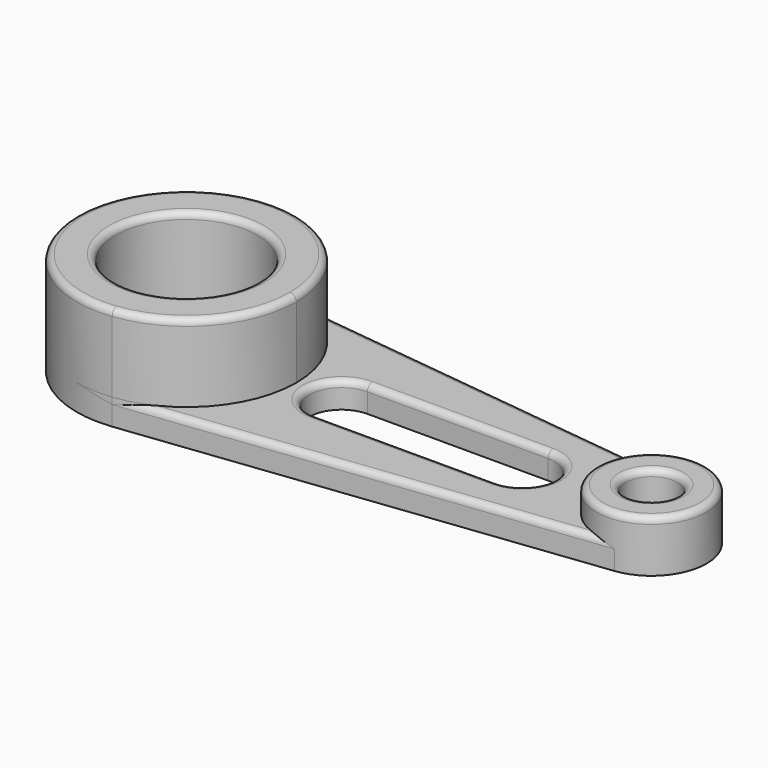
from build123d import *

# Parameters (mm, degrees)
F0_R         = 34.925
F1_DEPTH     = 50.8
F2_DEPTH     = 12.7
F0_R_2       = 12.7
F3_DEPTH     = 25.4
F4_F1_R      = 3.175
F4_F2_R      = 3.175
F4_F3_R      = 3.175
F4_F4_R      = 3.175
F4_F5_R      = 3.175
F4_T9_DEPTH  = 264.3151886434
F4_S10_R     = 27.051
F4_T11_DEPTH = 134
F4_S12_R     = 53.975
F4_T13_DEPTH = 134
F4_T17_DEPTH = 264.3151886434
F4_S18_R     = 27.051
F4_T19_DEPTH = 134
F4_S20_R     = 53.975
F4_T21_DEPTH = 134


# Not quite as in the source:
# - a fillet or chamfer that OpenCascade refuses, or shapes differently, is made with other operations: its cross-section is extruded or revolved along the edge and cut away or added


with BuildPart() as f1:
    # F0 (on Top) → F1 (new body)
    with BuildSketch(Plane.XY):
        with BuildLine():
            ThreePointArc((-174.625, 0), (-188.2488990323, 35.8481418723), (-222.2429444444, 53.5993327352))
            ThreePointArc((-222.2429444444, 53.5993327352), (-282.575, 0), (-222.2429444444, -53.5993327352))
            ThreePointArc((-222.2429444444, -53.5993327352), (-188.2488990323, -35.8481418723), (-174.625, 0))
        make_face()
        with Locations((-228.6, 0)):
            Circle(F0_R, mode=Mode.SUBTRACT)
    extrude(amount=F1_DEPTH)

    # F0 (on Top) → F2 (join)
    with BuildSketch(Plane.XY):
        with BuildLine():
            ThreePointArc((3.1860066667, -26.8627244061), (-27.051, 0), (3.1860066667, 26.8627244061))
            Line((3.1860066667, 26.8627244061), (-222.2429444444, 53.5993327352))
            ThreePointArc((-222.2429444444, 53.5993327352), (-188.2488990323, 35.8481418723), (-174.625, 0))
            ThreePointArc((-174.625, 0), (-188.2488990323, -35.8481418723), (-222.2429444444, -53.5993327352))
            Line((-222.2429444444, -53.5993327352), (3.1860066667, -26.8627244061))
        make_face()
        with BuildLine():
            ThreePointArc((-63.5, 15.875), (-52.2746798487, 11.2253201513), (-47.625, 0))
            ThreePointArc((-47.625, 0), (-52.2746798487, -11.2253201513), (-63.5, -15.875))
            Line((-63.5, -15.875), (-152.4, -15.875))
            ThreePointArc((-152.4, -15.875), (-168.275, 0), (-152.4, 15.875))
            Line((-152.4, 15.875), (-63.5, 15.875))
        make_face(mode=Mode.SUBTRACT)
    extrude(amount=F2_DEPTH)

    # F0 (on Top) → F3 (join)
    with BuildSketch(Plane.XY):
        with BuildLine():
            ThreePointArc((3.1860066667, -26.8627244061), (20.2230223673, -17.9662452207), (27.051, 0))
            ThreePointArc((27.051, 0), (20.2230223673, 17.9662452207), (3.1860066667, 26.8627244061))
            ThreePointArc((3.1860066667, 26.8627244061), (-27.051, 0), (3.1860066667, -26.8627244061))
        make_face()
        Circle(F0_R_2, mode=Mode.SUBTRACT)
    extrude(amount=F3_DEPTH)

    # F4: fillet of radius 3.175 on 10 edges, made by hand

    # F4_f1
    f4_f1_edges = [f1.edges().sort_by_distance(p)[0] for p in [
        (-234.9570555556, 53.5993327352, 50.8),
    ]]
    fillet(f4_f1_edges, radius=F4_F1_R)

    # F4_f2
    f4_f2_edges = [f1.edges().sort_by_distance(p)[0] for p in [
        (-47.625, 0, 12.7),
        (-107.95, -15.875, 12.7),
        (-168.275, 0, 12.7),
        (-107.95, 15.875, 12.7),
    ]]
    fillet(f4_f2_edges, radius=F4_F2_R)

    # F4_f3
    f4_f3_edges = [f1.edges().sort_by_distance(p)[0] for p in [
        (-263.525, 0, 50.8),
    ]]
    fillet(f4_f3_edges, radius=F4_F3_R)

    # F4_f4
    f4_f4_edges = [f1.edges().sort_by_distance(p)[0] for p in [
        (-3.1860066667, 26.8627244061, 25.4),
    ]]
    fillet(f4_f4_edges, radius=F4_F4_R)

    # F4_f5
    f4_f5_edges = [f1.edges().sort_by_distance(p)[0] for p in [
        (-12.7, 0, 25.4),
    ]]
    fillet(f4_f5_edges, radius=F4_F5_R)


with BuildPart() as f4_tool7:
    # F4_s8 → F4_t9 (new body)
    with BuildSketch(Plane(origin=(-249.0757155531, -29.5411916624, 0), x_dir=(0, 0, 1), z_dir=(0.9930399766, 0.1177777778, 0))):
        with BuildLine():
            ThreePointArc((12.7, 23.876), (11.7700640303, 26.1210640303), (9.525, 27.051))
            Line((9.525, 27.051), (9.525, 27.1145))
            Line((9.525, 27.1145), (12.7635, 27.1145))
            Line((12.7635, 27.1145), (12.7635, 23.876))
            Line((12.7635, 23.876), (12.7, 23.876))
        make_face()
    extrude(amount=F4_T9_DEPTH)

    # F4_s10 → F4_t11 (cut, symmetric)
    with BuildSketch(Plane.XY.offset(11.1)):
        Circle(F4_S10_R)
    extrude(amount=F4_T11_DEPTH, both=True, mode=Mode.SUBTRACT)

    # F4_s12 → F4_t13 (cut, symmetric)
    with BuildSketch(Plane.XY.offset(11.1)):
        with Locations((-228.6, 0)):
            Circle(F4_S12_R)
    extrude(amount=F4_T13_DEPTH, both=True, mode=Mode.SUBTRACT)


with BuildPart() as f1_1:
    add(f1.part)

    # F4_t6: cut F4_tool7
    add(f4_tool7.part, mode=Mode.SUBTRACT)


with BuildPart() as f4_tool15:
    # F4_s16 → F4_t17 (new body)
    with BuildSketch(Plane(origin=(13.3998331838, -1.5892638889, 0), x_dir=(0, 0, 1), z_dir=(-0.9930399766, 0.1177777778, 0))):
        with BuildLine():
            ThreePointArc((9.525, 27.051), (11.7700640303, 26.1210640303), (12.7, 23.876))
            Line((12.7, 23.876), (12.7635, 23.876))
            Line((12.7635, 23.876), (12.7635, 27.1145))
            Line((12.7635, 27.1145), (9.525, 27.1145))
            Line((9.525, 27.1145), (9.525, 27.051))
        make_face()
    extrude(amount=F4_T17_DEPTH)

    # F4_s18 → F4_t19 (cut, symmetric)
    with BuildSketch(Plane.XY.offset(11.1)):
        Circle(F4_S18_R)
    extrude(amount=F4_T19_DEPTH, both=True, mode=Mode.SUBTRACT)

    # F4_s20 → F4_t21 (cut, symmetric)
    with BuildSketch(Plane.XY.offset(11.1)):
        with Locations((-228.6, 0)):
            Circle(F4_S20_R)
    extrude(amount=F4_T21_DEPTH, both=True, mode=Mode.SUBTRACT)


with BuildPart() as f1_2:
    add(f1_1.part)

    # F4_t14: cut F4_tool15
    add(f4_tool15.part, mode=Mode.SUBTRACT)


solid = f1_2.part
